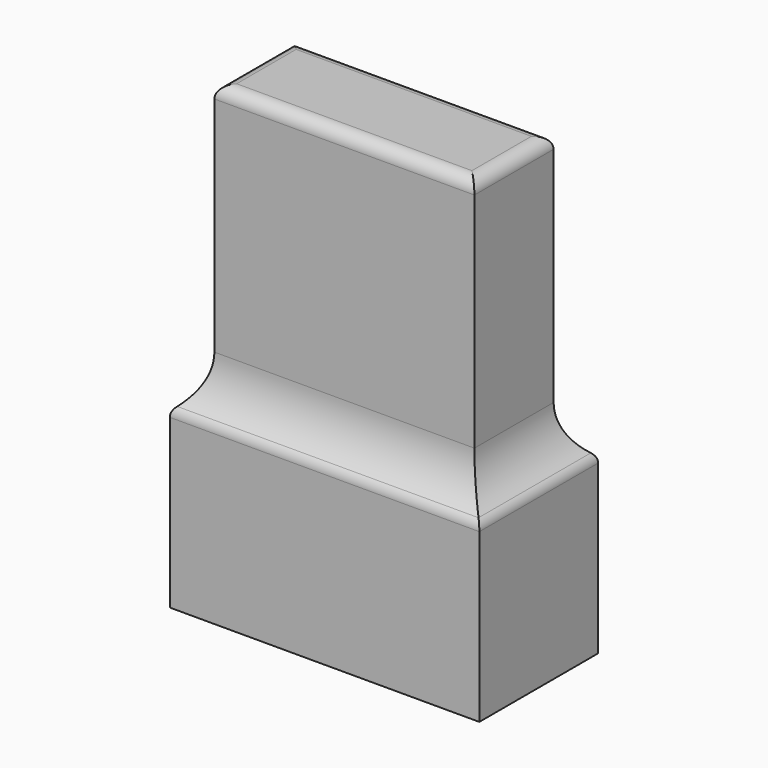
from build123d import *

# Parameters (mm, degrees)
F0_W           = 25
F0_H           = 12
F0_W_2         = 19
F0_H_2         = 8
F1_DEPTH       = 10
F2_W           = 21
F2_H           = 8
F2_W_2         = 17
F2_H_2         = 2
F3_DEPTH       = 25
F4_W           = 21
F4_H           = 8
F4_W_2         = 17
F4_H_2         = 2
F5_DEPTH       = 2
F6_W           = 25
F6_H           = 12
F7_DEPTH       = 4
F10_DEPTH      = 4
F10_DEPTH_BACK = 4
F11_T1_DEPTH   = 21
F11_T3_DEPTH   = 8
F11_T9_DEPTH   = 31
F11_T14_DEPTH  = 18
F11_T22_DEPTH  = 31
F11_T27_DEPTH  = 18
F11_T35_DEPTH  = 31
F11_T40_DEPTH  = 18
F11_T48_DEPTH  = 18
F11_T53_DEPTH  = 31
F12_R          = 1
F14_DEPTH      = 1


# Not quite as in the source:
# - a fillet or chamfer that OpenCascade refuses, or shapes differently, is made with other operations: its cross-section is extruded or revolved along the edge and cut away or added


with BuildPart() as f1:
    # F0 (on Top) → F1 (new body)
    with BuildSketch(Plane.XY):
        with Locations((12.5, 6)):
            Rectangle(F0_W, F0_H)
        with Locations((12.5, 6)):
            Rectangle(F0_W_2, F0_H_2, mode=Mode.SUBTRACT)
    extrude(amount=-F1_DEPTH)

    # F2 (on Top) → F3 (join)
    with BuildSketch(Plane.XY):
        with Locations((12.5, 6)):
            Rectangle(F2_W, F2_H)
        with Locations((12.5, 6)):
            Rectangle(F2_W_2, F2_H_2, mode=Mode.SUBTRACT)
    extrude(amount=F3_DEPTH)

    # F4 (on face) → F5 (join)
    with BuildSketch(Plane.XY.offset(25)):
        with Locations((12.5, 6)):
            Rectangle(F4_W, F4_H)
        with Locations((12.5, 6)):
            Rectangle(F4_W_2, F4_H_2, mode=Mode.SUBTRACT)
        with Locations((12.5, 6)):
            Rectangle(F4_W_2, F4_H_2)
    extrude(amount=F5_DEPTH)

    # F6 (on face) → F7 (join)
    with BuildSketch(Plane.XY):
        with Locations((12.5, 6)):
            Rectangle(F6_W, F6_H)
        Polygon((23, 2), (22, 2), (3, 2), (2, 2), (2, 10), (3, 10), (22, 10), (23, 10), align=None, mode=Mode.SUBTRACT)
    extrude(amount=F7_DEPTH)

    # F9 (on offset) → F10 (join, two sides)
    with BuildSketch(Plane.XZ.offset(-6)) as f10_sk:
        with BuildLine():
            Line((3, -7), (3, -8.5))
            Line((3, -8.5), (3.4671572875, -8.0328427125))
            ThreePointArc((3.4671572875, -8.0328427125), (3.5843145751, -7.75), (3.4671572875, -7.4671572875))
            Line((3.4671572875, -7.4671572875), (3, -7))
        make_face()
        with BuildLine():
            Line((21.5328427125, -8.0328427125), (22, -8.5))
            Line((22, -8.5), (22, -7))
            Line((22, -7), (21.5328427125, -7.4671572875))
            ThreePointArc((21.5328427125, -7.4671572875), (21.4156854249, -7.75), (21.5328427125, -8.0328427125))
        make_face()
    extrude(amount=F10_DEPTH)
    extrude(f10_sk.sketch, amount=-F10_DEPTH_BACK)

    # F11: fillet of radius 5 on 4 edges, made by hand

    # F11_s2 → F11_t1 (join)
    with BuildSketch(Plane.YZ.offset(2)):
        with BuildLine():
            ThreePointArc((0, 4), (1.472135955, 5.7639320225), (2, 8))
            Line((2, 8), (2, 4))
            Line((2, 4), (0, 4))
        make_face()
        with BuildLine():
            ThreePointArc((12, 4), (10.527864045, 5.7639320225), (10, 8))
            Line((10, 8), (10, 4))
            Line((10, 4), (12, 4))
        make_face()
    extrude(amount=F11_T1_DEPTH)

    # F11_s4 → F11_t3 (join)
    with BuildSketch(Plane.XZ.offset(-10)):
        with BuildLine():
            ThreePointArc((25, 4), (23.527864045, 5.7639320225), (23, 8))
            Line((23, 8), (23, 4))
            Line((23, 4), (25, 4))
        make_face()
        with BuildLine():
            ThreePointArc((0, 4), (1.472135955, 5.7639320225), (2, 8))
            Line((2, 8), (2, 4))
            Line((2, 4), (0, 4))
        make_face()
    extrude(amount=F11_T3_DEPTH)


with BuildPart() as f11_tool7:
    # F11_s8 → F11_t9 (new body)
    with BuildSketch(Plane.YZ.offset(-8)):
        with BuildLine():
            ThreePointArc((0, 4), (1.472135955, 5.7639320225), (2, 8))
            Line((2, 8), (2, 4))
            Line((2, 4), (0, 4))
        make_face()
    extrude(amount=F11_T9_DEPTH)

    split(bisect_by=Plane.YZ, keep=Keep.TOP)

    split(bisect_by=Plane.YZ.offset(2), keep=Keep.BOTTOM)


with BuildPart() as f11_tool12:
    # F11_s13 → F11_t14 (new body)
    with BuildSketch(Plane.XZ.offset(8)):
        with BuildLine():
            ThreePointArc((0, 4), (1.472135955, 5.7639320225), (2, 8))
            Line((2, 8), (2, 4))
            Line((2, 4), (0, 4))
        make_face()
    extrude(amount=-F11_T14_DEPTH)

    split(bisect_by=Plane.XZ, keep=Keep.BOTTOM)

    split(bisect_by=Plane.XZ.offset(-2), keep=Keep.TOP)


with BuildPart() as f11_tool7_1:
    add(f11_tool7.part)

    # F11_t17: intersect F11_tool12
    add(f11_tool12.part, mode=Mode.INTERSECT)


with BuildPart() as f1_1:
    add(f1.part)

    # F11_t5: union F11_tool7
    add(f11_tool7_1.part)


with BuildPart() as f11_tool20:
    # F11_s21 → F11_t22 (new body)
    with BuildSketch(Plane.YZ.offset(2)):
        with BuildLine():
            ThreePointArc((0, 4), (1.472135955, 5.7639320225), (2, 8))
            Line((2, 8), (2, 4))
            Line((2, 4), (0, 4))
        make_face()
    extrude(amount=F11_T22_DEPTH)

    split(bisect_by=Plane.YZ.offset(25), keep=Keep.BOTTOM)

    split(bisect_by=Plane.YZ.offset(23), keep=Keep.TOP)


with BuildPart() as f11_tool25:
    # F11_s26 → F11_t27 (new body)
    with BuildSketch(Plane.XZ.offset(-10)):
        with BuildLine():
            ThreePointArc((25, 4), (23.527864045, 5.7639320225), (23, 8))
            Line((23, 8), (23, 4))
            Line((23, 4), (25, 4))
        make_face()
    extrude(amount=F11_T27_DEPTH)

    split(bisect_by=Plane.XZ, keep=Keep.BOTTOM)

    split(bisect_by=Plane.XZ.offset(-2), keep=Keep.TOP)


with BuildPart() as f11_tool20_1:
    add(f11_tool20.part)

    # F11_t30: intersect F11_tool25
    add(f11_tool25.part, mode=Mode.INTERSECT)


with BuildPart() as f1_2:
    add(f1_1.part)

    # F11_t18: union F11_tool20
    add(f11_tool20_1.part)


with BuildPart() as f11_tool33:
    # F11_s34 → F11_t35 (new body)
    with BuildSketch(Plane.YZ.offset(33)):
        with BuildLine():
            ThreePointArc((12, 4), (10.527864045, 5.7639320225), (10, 8))
            Line((10, 8), (10, 4))
            Line((10, 4), (12, 4))
        make_face()
    extrude(amount=-F11_T35_DEPTH)

    split(bisect_by=Plane.YZ.offset(25), keep=Keep.BOTTOM)

    split(bisect_by=Plane.YZ.offset(23), keep=Keep.TOP)


with BuildPart() as f11_tool38:
    # F11_s39 → F11_t40 (new body)
    with BuildSketch(Plane.XZ.offset(-20)):
        with BuildLine():
            ThreePointArc((25, 4), (23.527864045, 5.7639320225), (23, 8))
            Line((23, 8), (23, 4))
            Line((23, 4), (25, 4))
        make_face()
    extrude(amount=F11_T40_DEPTH)

    split(bisect_by=Plane.XZ.offset(-12), keep=Keep.TOP)

    split(bisect_by=Plane.XZ.offset(-10), keep=Keep.BOTTOM)


with BuildPart() as f11_tool33_1:
    add(f11_tool33.part)

    # F11_t43: intersect F11_tool38
    add(f11_tool38.part, mode=Mode.INTERSECT)


with BuildPart() as f1_3:
    add(f1_2.part)

    # F11_t31: union F11_tool33
    add(f11_tool33_1.part)


with BuildPart() as f11_tool46:
    # F11_s47 → F11_t48 (new body)
    with BuildSketch(Plane.XZ.offset(-2)):
        with BuildLine():
            ThreePointArc((0, 4), (1.472135955, 5.7639320225), (2, 8))
            Line((2, 8), (2, 4))
            Line((2, 4), (0, 4))
        make_face()
    extrude(amount=-F11_T48_DEPTH)

    split(bisect_by=Plane.XZ.offset(-12), keep=Keep.TOP)

    split(bisect_by=Plane.XZ.offset(-10), keep=Keep.BOTTOM)


with BuildPart() as f11_tool51:
    # F11_s52 → F11_t53 (new body)
    with BuildSketch(Plane.YZ.offset(23)):
        with BuildLine():
            ThreePointArc((12, 4), (10.527864045, 5.7639320225), (10, 8))
            Line((10, 8), (10, 4))
            Line((10, 4), (12, 4))
        make_face()
    extrude(amount=-F11_T53_DEPTH)

    split(bisect_by=Plane.YZ, keep=Keep.TOP)

    split(bisect_by=Plane.YZ.offset(2), keep=Keep.BOTTOM)


with BuildPart() as f11_tool46_1:
    add(f11_tool46.part)

    # F11_t56: intersect F11_tool51
    add(f11_tool51.part, mode=Mode.INTERSECT)


with BuildPart() as f1_4:
    add(f1_3.part)

    # F11_t44: union F11_tool46
    add(f11_tool46_1.part)

    # F12
    f12_edges = [f1_4.edges().sort_by_distance(p)[0] for p in [
        (23, 6, 27),
        (12.5, 2, 27),
        (2, 6, 27),
        (12.5, 10, 27),
        (12.5, 12, 4),
        (25, 6, 4),
        (12.5, 0, 4),
        (0, 6, 4),
    ]]
    fillet(f12_edges, radius=F12_R)

    # F13 (on face) → F14 (cut)
    with BuildSketch(Plane(origin=(0, 10, 0), x_dir=(-1, 0, 0), z_dir=(0, 1, 0))):
        Polygon((-12.5, 20.9), (-17, 13.1057713659), (-8, 13.1057713659), align=None)
        with BuildLine():
            Line((-12.75, 13.6057713659), (-16.1339745962, 13.6057713659))
            Line((-16.1339745962, 13.6057713659), (-14.4419872981, 16.536379332))
            Line((-14.4419872981, 16.536379332), (-14.4290420842, 16.5289054093))
            ThreePointArc((-14.4290420842, 16.5289054093), (-14.3169872981, 14.6548094716), (-12.75, 13.6207192114))
            Line((-12.75, 13.6207192114), (-12.75, 13.6057713659))
        make_face(mode=Mode.SUBTRACT)
        with BuildLine():
            ThreePointArc((-12.75, 14.125447255), (-14.0980762114, 15.7038475773), (-12.75, 17.2822478995))
            Line((-12.75, 17.2822478995), (-12.75, 14.125447255))
        make_face(mode=Mode.SUBTRACT)
        with BuildLine():
            ThreePointArc((-12.25, 17.2822478995), (-10.9019237886, 15.7038475773), (-12.25, 14.125447255))
            Line((-12.25, 14.125447255), (-12.25, 17.2822478995))
        make_face(mode=Mode.SUBTRACT)
        with BuildLine():
            Line((-8.8660254038, 13.6057713659), (-12.25, 13.6057713659))
            Line((-12.25, 13.6057713659), (-12.25, 13.6207192114))
            ThreePointArc((-12.25, 13.6207192114), (-10.6830127019, 14.6548094716), (-10.5709579158, 16.5289054093))
            Line((-10.5709579158, 16.5289054093), (-10.5580127019, 16.536379332))
            Line((-10.5580127019, 16.536379332), (-8.8660254038, 13.6057713659))
        make_face(mode=Mode.SUBTRACT)
        with BuildLine():
            Line((-12.75, 19.4669872981), (-12.75, 17.7869759432))
            ThreePointArc((-12.75, 17.7869759432), (-13.5490381057, 17.5208348754), (-14.1790420842, 16.9619181112))
            Line((-14.1790420842, 16.9619181112), (-14.1919872981, 16.9693920339))
            Line((-14.1919872981, 16.9693920339), (-12.75, 19.4669872981))
        make_face(mode=Mode.SUBTRACT)
        with BuildLine():
            Line((-12.25, 17.7869759432), (-12.25, 19.4669872981))
            Line((-12.25, 19.4669872981), (-10.8080127019, 16.9693920339))
            Line((-10.8080127019, 16.9693920339), (-10.8209579158, 16.9619181112))
            ThreePointArc((-10.8209579158, 16.9619181112), (-11.4509618943, 17.5208348754), (-12.25, 17.7869759432))
        make_face(mode=Mode.SUBTRACT)
    extrude(amount=-F14_DEPTH, mode=Mode.SUBTRACT)


solid = f1_4.part
